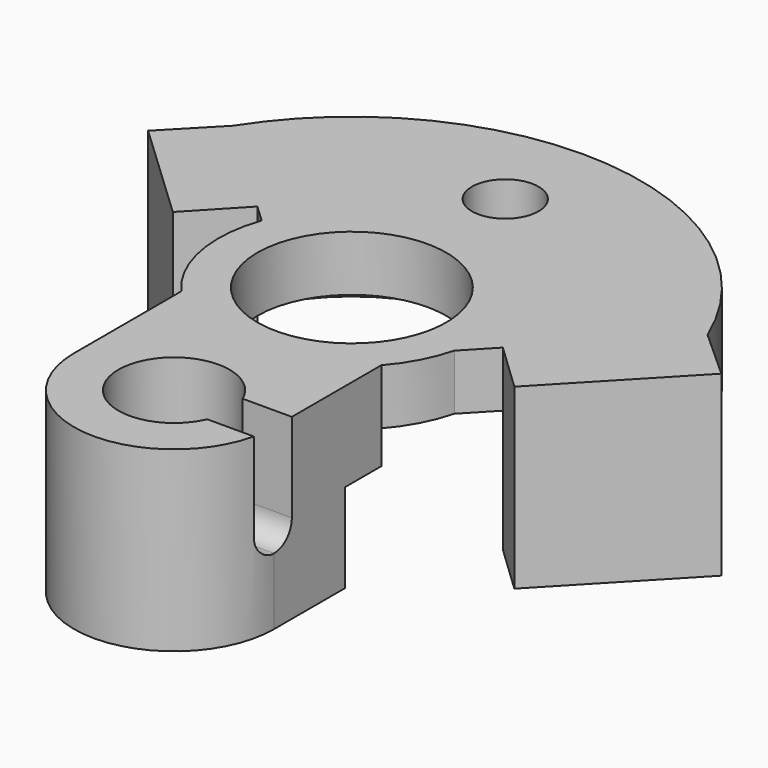
from build123d import *

# Parameters (mm, degrees)
F0_R          = 2.5
F1_DEPTH      = 4
F2_DEPTH      = 4
F4_DEPTH      = 4
F4_DEPTH_BACK = 4
F5_DEPTH      = 1.5
F6_D          = 8.5
F8_DEPTH      = 5
F9_R          = 1
F11_D         = 3


# Not quite as in the source:
# - a feature names something its author has since deleted; it is built from what else it names


with BuildPart() as f1:
    # F0 (on Top) → F1 (new body)
    with BuildSketch(Plane.XY):
        with BuildLine():
            ThreePointArc((-5.6568542495, 2), (1.7516630026, 5.7386127875), (5.8094750193, -1.5))
            Line((5.8094750193, -1.5), (12, 5))
            ThreePointArc((12, 5), (1.1284028976, 12.9509345956), (-10.9544511501, 7))
            Line((-10.9544511501, 7), (-5.6568542495, 2))
        make_face()
        with BuildLine():
            Line((-3.3166247904, -5), (3.3166247904, -5))
            ThreePointArc((3.3166247904, -5), (3.9421870024, -4.5231804782), (4.5, -3.9686269666))
            ThreePointArc((4.5, -3.9686269666), (5.3004573924, -2.8116101137), (5.8094750193, -1.5))
            ThreePointArc((5.8094750193, -1.5), (1.7516630026, 5.7386127875), (-5.6568542495, 2))
            ThreePointArc((-5.6568542495, 2), (-5.8903776643, -1.1416877735), (-4.5, -3.9686269666))
            ThreePointArc((-4.5, -3.9686269666), (-3.9421870024, -4.5231804782), (-3.3166247904, -5))
        make_face()
        with BuildLine():
            ThreePointArc((4.5, -3.9686269666), (3.9421870024, -4.5231804782), (3.3166247904, -5))
            Line((3.3166247904, -5), (-3.3166247904, -5))
            ThreePointArc((-3.3166247904, -5), (-3.9421870024, -4.5231804782), (-4.5, -3.9686269666))
            Line((-4.5, -3.9686269666), (-4.5, -6))
            Line((-4.5, -6), (4.5, -6))
            Line((4.5, -6), (4.5, -3.9686269666))
        make_face()
        with BuildLine():
            Line((4.5, -10), (4.5, -6))
            Line((4.5, -6), (-4.5, -6))
            Line((-4.5, -6), (-4.5, -10))
            ThreePointArc((-4.5, -10), (0, -14.5), (4.5, -10))
        make_face()
        with Locations((0, -10)):
            Circle(F0_R, mode=Mode.SUBTRACT)
    extrude(amount=F1_DEPTH)

    # F0 (on Top) → F2 (join)
    with BuildSketch(Plane.XY):
        with BuildLine():
            Line((4.5, -10), (4.5, -6))
            Line((4.5, -6), (-4.5, -6))
            Line((-4.5, -6), (-4.5, -10))
            ThreePointArc((-4.5, -10), (0, -14.5), (4.5, -10))
        make_face()
        with Locations((0, -10)):
            Circle(F0_R, mode=Mode.SUBTRACT)
    extrude(amount=-F2_DEPTH)

    # F3 (on face) → F4 (join, two sides)
    with BuildSketch(Plane.XY) as f4_sk:
        Polygon((6.9953599884, -0.2548305963), (9.1677656379, -2.3238046642), (14.2284593947, 2.9898819005), (12, 5), align=None)
        Polygon((-8.5004540069, 0.5586628434), (-6.4412987824, 2.7403777105), (-10.9544511501, 7), (-13.0414362661, 4.8445516572), align=None)
    extrude(amount=-F4_DEPTH)
    extrude(f4_sk.sketch, amount=F4_DEPTH_BACK)

    # F3 (on face) → F5 (cut)
    with BuildSketch(Plane.XY):
        with BuildLine():
            Line((5.8094750193, -1.5), (6.9953599884, -0.2548305963))
            ThreePointArc((6.9953599884, -0.2548305963), (1.5230115414, 6.832308237), (-6.4412987824, 2.7403777105))
            Line((-6.4412987824, 2.7403777105), (-5.6568542495, 2))
            ThreePointArc((-5.6568542495, 2), (1.7516630026, 5.7386127875), (5.8094750193, -1.5))
        make_face()
        with BuildLine():
            ThreePointArc((4.5, -3.9686269666), (5.3004573924, -2.8116101137), (5.8094750193, -1.5))
            ThreePointArc((5.8094750193, -1.5), (1.7516630026, 5.7386127875), (-5.6568542495, 2))
            ThreePointArc((-5.6568542495, 2), (-5.8903776643, -1.1416877735), (-4.5, -3.9686269666))
            ThreePointArc((-4.5, -3.9686269666), (-3.9421870024, -4.5231804782), (-3.3166247904, -5))
            Line((-3.3166247904, -5), (3.3166247904, -5))
            ThreePointArc((3.3166247904, -5), (3.9421870024, -4.5231804782), (4.5, -3.9686269666))
        make_face()
    extrude(amount=F5_DEPTH, mode=Mode.SUBTRACT)

    # F6 (through all)
    with Locations(Plane(origin=(0, 0, 0), x_dir=(1, 0, 0), z_dir=(0, 0, -1))):
        with Locations((0, 0)):
            Hole(F6_D / 2)

    # F7 (on face) → F8 (cut)
    with BuildSketch(Plane.XY.offset(4)):
        with BuildLine():
            Line((4.5, -9), (2.2912878475, -9))
            ThreePointArc((2.2912878475, -9), (2.4472657823, -9.4892258908), (2.5, -10))
            ThreePointArc((2.5, -10), (2.4472657823, -10.5107741092), (2.2912878475, -11))
            Line((2.2912878475, -11), (4.3874821937, -11))
            ThreePointArc((4.3874821937, -11), (4.4717820761, -10.5031551095), (4.5, -10))
            Line((4.5, -10), (4.5, -9))
        make_face()
    extrude(amount=-F8_DEPTH, mode=Mode.SUBTRACT)

    # F9
    f9_edges = [f1.edges().sort_by_distance(p)[0] for p in [
        (3.339385, -11, -1),
        (3.395644, -9, -1),
    ]]
    fillet(f9_edges, radius=F9_R)

    # F11 (through all)
    with Locations(Plane.XY.offset(4)):
        with Locations((0, 8.625)):
            Hole(F11_D / 2)


solid = f1.part
